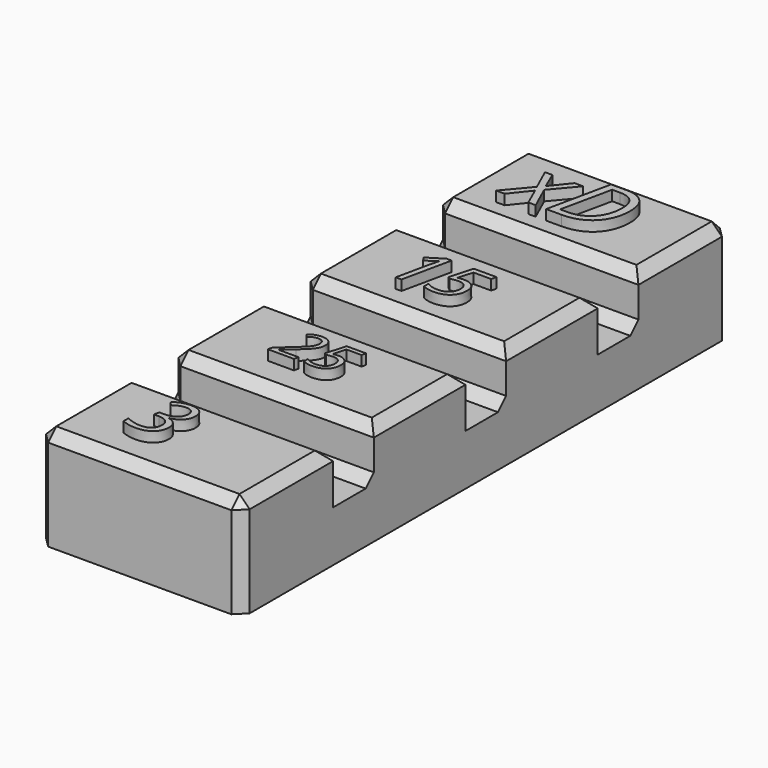
from build123d import *

# Parameters (mm, degrees)
F0_W          = 25.4
F0_H          = 76.2
F1_DEPTH      = 12.7
F2_W          = 6.35
F2_H          = 12.7
F3_DEPTH      = 25.401
F4_SIZE       = 1.27
F5_T          = 2.54
F5_T3_DEPTH   = 6.8760512242
F5_T5_DEPTH   = 6.8760512242
F5_T7_DEPTH   = 29.21
F5_T9_DEPTH   = 6.8760512242
F5_T11_DEPTH  = 6.8760512242
F6_TEXT_SIZE  = 9.6655773068
F7_DEPTH      = 1.27
F8_TEXT_SIZE  = 7.424920073
F9_DEPTH      = 1.27
F10_TEXT_SIZE = 8.6505942616
F11_DEPTH     = 1.27
F12_TEXT_SIZE = 11.226358927
F13_DEPTH     = 1.27


# Not quite as in the source:
# - a shell that OpenCascade refuses in one call is made with other operations: the cavity is built on its own and cut out
# - Text() gives the source's letters only with a copy of the font that has no kerning and outlines rounded to 1/6400 em; it was checked with that copy


with BuildPart() as f1:
    # F0 (on Top) → F1 (new body)
    with BuildSketch(Plane.XY):
        Rectangle(F0_W, F0_H)
    extrude(amount=F1_DEPTH)

    # F2 (on face) → F3 (cut, through all)
    with BuildSketch(Plane(origin=(-12.7, 0, 0), x_dir=(0, -1, 0), z_dir=(-1, 0, 0))):
        with Locations((0, 12.7)):
            Rectangle(F2_W, F2_H)
        with Locations((20.6375, 12.7)):
            Rectangle(F2_W, F2_H)
        with Locations((-20.6375, 12.7)):
            Rectangle(F2_W, F2_H)
    extrude(amount=-F3_DEPTH, mode=Mode.SUBTRACT)

    # F4
    f4_edges = [f1.edges().sort_by_distance(p)[0] for p in [
        (0, 38.1, 12.7),
        (12.7, 30.95625, 12.7),
        (0, 23.8125, 12.7),
        (-12.7, 30.95625, 12.7),
        (0, 17.4625, 12.7),
        (12.7, 10.31875, 12.7),
        (0, 3.175, 12.7),
        (-12.7, 10.31875, 12.7),
        (0, -3.175, 12.7),
        (12.7, -10.31875, 12.7),
        (0, -17.4625, 12.7),
        (-12.7, -10.31875, 12.7),
        (0, -38.1, 12.7),
        (0, -23.8125, 12.7),
        (12.7, -30.95625, 12.7),
        (-12.7, -30.95625, 12.7),
        (0, 23.8125, 6.35),
        (-12.7, 0, 6.35),
        (-12.7, -20.6375, 6.35),
        (-12.7, 20.6375, 6.35),
        (0, 3.175, 6.35),
        (0, -17.4625, 6.35),
        (-12.7, 38.1, 6.35),
        (-12.7, -38.1, 6.35),
        (12.7, -38.1, 6.35),
        (12.7, 38.1, 6.35),
        (-12.7, -17.4625, 9.525),
        (-12.7, 3.175, 9.525),
        (-12.7, 23.8125, 9.525),
    ]]
    chamfer(f4_edges, length=F4_SIZE)

    # F5: shell of thickness 2.54, made by hand


with BuildPart() as f5_core1:
    # F5_t2: copy of F1
    add(f1.part)

    # the walls: a layer under each face that stays
    f5_faces = [f5_core1.faces().sort_by_distance(p)[0] for p in [
        (-12.7, 24.5533333333, 5.715),
        (-12.065, 37.465, 5.715),
        (-12.065, -37.465, 5.715),
        (-12.065, 30.95625, 12.065),
        (-12.065, -30.32125, 12.065),
        (-12.065, 24.4475, 9.525),
        (0, -23.8125, 8.255),
        (-12.065, 23.495, 6.6675),
        (-12.065, 20.0025, 5.715),
        (-12.065, -21.2725, 5.715),
        (0, 17.4625, 8.255),
        (-12.065, -17.78, 6.6675),
        (-12.065, -16.8275, 9.525),
        (-12.065, 10.95375, 12.065),
        (-12.065, -9.68375, 12.065),
        (-12.065, 3.81, 9.525),
        (0, -3.175, 8.255),
        (-12.065, 2.8575, 6.6675),
        (-12.065, -0.635, 5.715),
        (0, 38.1, 5.715),
        (0, -38.1, 5.715),
        (12.065, 37.465, 5.715),
        (12.065, -37.465, 5.715),
        (12.7, 0, 5.715),
        (-12.065, 37.1475, 11.7475),
        (-12.065, -37.1475, 11.7475),
        (0, 30.95625, 12.7),
        (-12.065, 24.765, 11.7475),
        (0, -24.4475, 12.065),
        (0, -30.95625, 12.7),
        (0.635, 23.8125, 9.525),
        (0.635, -21.2725, 6.35),
        (0.635, 23.1775, 6.985),
        (0.635, 20.0025, 6.35),
        (0, 16.8275, 12.065),
        (0.635, -18.0975, 6.985),
        (-12.065, -16.51, 11.7475),
        (0.635, -17.4625, 9.525),
        (0, 10.31875, 12.7),
        (-12.065, 4.1275, 11.7475),
        (0, -3.81, 12.065),
        (0, -10.31875, 12.7),
        (0.635, 3.175, 9.525),
        (0.635, -0.635, 6.35),
        (0.635, 2.54, 6.985),
        (0, 37.465, 12.065),
        (0, -37.465, 12.065),
        (12.065, 37.1475, 11.7475),
        (12.065, -37.1475, 11.7475),
        (12.065, -30.32125, 12.065),
        (12.065, 30.32125, 12.065),
        (12.065, -10.31875, 12.065),
        (12.065, 10.31875, 12.065),
        (0.635, 24.4475, 12.065),
        (0.635, -16.8275, 12.065),
        (0.635, 3.81, 12.065),
    ]]
    thicken(f5_faces, amount=-F5_T, mode=Mode.SUBTRACT)

    # F5_s4 → F5_t3 (cut)
    with BuildSketch(Plane(origin=(-20.6873012242, 20.6873012242, 0), x_dir=(0, 0, 1), z_dir=(0.7071067812, -0.7071067812, 0))):
        Polygon((7.6346646968, -8.7096107049), (7.62, -11.295749718), (6.8126933972, -11.295749718), (6.1535303163, -10.8296510336), align=None)
    extrude(amount=F5_T3_DEPTH, mode=Mode.SUBTRACT)

    # F5_s6 → F5_t5 (cut)
    with BuildSketch(Plane(origin=(-5.6060512242, 0, -5.6060512242), x_dir=(0, 1, 0), z_dir=(0.7071067812, 0, 0.7071067812))):
        Polygon((-23.7871, 12.5977585695), (-26.3525, 12.5723585695), (-26.3525, 10.0323585695), (-23.8125, 10.0323585695), align=None)
        Polygon((22.5278353032, 12.6184975827), (24.0089696837, 10.4984572539), (23.3498066028, 10.0323585695), (22.5425, 10.0323585695), align=None)
        Polygon((17.4879, 12.5977585695), (17.4625, 10.0323585695), (14.9225, 10.0323585695), (14.9225, 12.5723585695), align=None)
        Polygon((-18.7471646968, 12.6184975827), (-18.7325, 10.0323585695), (-17.9251933972, 10.0323585695), (-17.2660303163, 10.4984572539), align=None)
        Polygon((-3.1496, 12.5977585695), (-5.715, 12.5723585695), (-5.715, 10.0323585695), (-3.175, 10.0323585695), align=None)
        Polygon((1.8903353032, 12.6184975827), (3.3714696837, 10.4984572539), (2.7123066028, 10.0323585695), (1.905, 10.0323585695), align=None)
    extrude(amount=F5_T5_DEPTH, mode=Mode.SUBTRACT)

    # F5_s8 → F5_t7 (cut)
    with BuildSketch(Plane.YZ.offset(-13.97)):
        Polygon((-23.7871, 6.3754), (-26.3525, 6.35), (-26.3525, 3.81), (-23.8125, 3.81), align=None)
        Polygon((17.4879, 6.3754), (14.9225, 6.35), (14.9225, 3.81), (17.4625, 3.81), align=None)
        Polygon((-3.1496, 6.3754), (-5.715, 6.35), (-5.715, 3.81), (-3.175, 3.81), align=None)
        Polygon((23.7691394878, 7.6379605122), (26.3525, 7.62), (26.3525, 6.5678975516), (25.6085512242, 5.8239487758), align=None)
        Polygon((-18.7504605122, 6.3933605122), (-18.7325, 3.81), (-17.6803975516, 3.81), (-16.9364487758, 4.5539487758), align=None)
        Polygon((22.5245394878, 6.3933605122), (24.3385512242, 4.5539487758), (23.5946024484, 3.81), (22.5425, 3.81), align=None)
        Polygon((-17.5058605122, 7.6379605122), (-15.6664487758, 5.8239487758), (-14.9225, 6.5678975516), (-14.9225, 7.62), align=None)
        Polygon((3.1316394878, 7.6379605122), (5.715, 7.62), (5.715, 6.5678975516), (4.9710512242, 5.8239487758), align=None)
        Polygon((1.8870394878, 6.3933605122), (1.905, 3.81), (2.9571024484, 3.81), (3.7010512242, 4.5539487758), align=None)
    extrude(amount=F5_T7_DEPTH, mode=Mode.SUBTRACT)

    # F5_s10 → F5_t9 (cut)
    with BuildSketch(Plane(origin=(-0.0498012242, 0.0498012242, 0), x_dir=(0, 0, 1), z_dir=(0.7071067812, -0.7071067812, 0))):
        Polygon((7.6346646968, 20.4762216886), (6.1535303163, 18.3561813599), (6.8126933972, 17.8900826754), (7.62, 17.8900826754), align=None)
    extrude(amount=F5_T9_DEPTH, mode=Mode.SUBTRACT)

    # F5_s12 → F5_t11 (cut)
    with BuildSketch(Plane(origin=(-10.3685512242, 10.3685512242, 0), x_dir=(0, 0, 1), z_dir=(0.7071067812, -0.7071067812, 0))):
        Polygon((7.6346646968, 5.8833054919), (7.62, 3.2971664787), (6.8126933972, 3.2971664787), (6.1535303163, 3.7632651631), align=None)
    extrude(amount=F5_T11_DEPTH, mode=Mode.SUBTRACT)


with BuildPart() as f1_1:
    add(f1.part)

    # what is left inside the walls is the cavity
    f5_cavity = [f5_core1.part.solids().sort_by_distance(p)[0] for p in [
        (0, -11.853333, 0.0254),
    ]]
    add(f5_cavity, mode=Mode.SUBTRACT)

    # F6 (on face) → F7 (join)
    with BuildSketch(Plane.XY.offset(12.7)):
        with Locations((-5.6906086394, -34.0685312798)):
            Text('3', F6_TEXT_SIZE, font='Open Sans', font_style=FontStyle.ITALIC, text_align=(TextAlign.LEFT, TextAlign.BOTTOM))
    extrude(amount=F7_DEPTH)

    # F8 (on face) → F9 (join)
    with BuildSketch(Plane.XY.offset(12.7)):
        with Locations((-4.0095777949, -13.1603758782)):
            Text('25', F8_TEXT_SIZE, font='Open Sans', font_style=FontStyle.ITALIC, text_align=(TextAlign.LEFT, TextAlign.BOTTOM))
    extrude(amount=F9_DEPTH)

    # F10 (on face) → F11 (join)
    with BuildSketch(Plane.XY.offset(12.7)):
        with Locations((-5.4780161008, 6.4722741954)):
            Text('15', F10_TEXT_SIZE, font='Open Sans', font_style=FontStyle.ITALIC, text_align=(TextAlign.LEFT, TextAlign.BOTTOM))
    extrude(amount=F11_DEPTH)

    # F12 (on face) → F13 (join)
    with BuildSketch(Plane.XY.offset(12.7)):
        with Locations((-7.107175421, 26.8750861287)):
            Text('xD', F12_TEXT_SIZE, font='Open Sans', font_style=FontStyle.ITALIC, text_align=(TextAlign.LEFT, TextAlign.BOTTOM))
    extrude(amount=F13_DEPTH)


solid = f1_1.part
